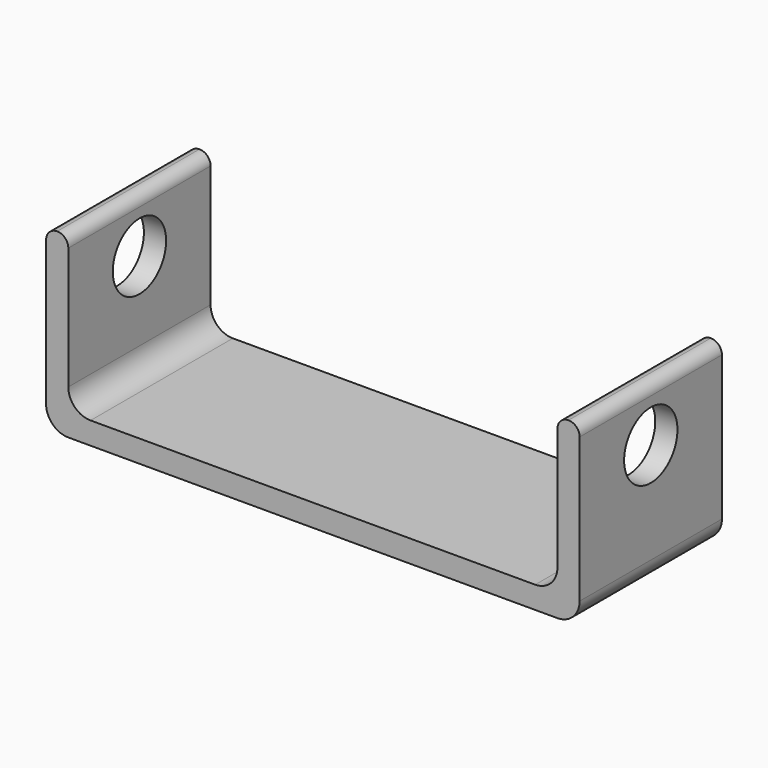
from build123d import *

# Parameters (mm, degrees)
F1_DEPTH = 25.4
F2_R     = 6.35
F3_R     = 3.17499
F4_R     = 9.525
F5_DEPTH = 152.401


# Not quite as in the source:
# - a fillet or chamfer is up to 0.001 mm smaller than in the source, because OpenCascade refuses the exact size


with BuildPart() as f1:
    # F0 (on Front) → F1 (new body, symmetric)
    with BuildSketch(Plane.XZ):
        Polygon((-76.2, 0), (0, 0), (76.2, 0), (76.2, 50.8), (69.85, 50.8), (69.85, 6.35), (0, 6.35), (-69.85, 6.35), (-69.85, 50.8), (-76.2, 50.8), align=None)
    extrude(amount=F1_DEPTH, both=True)

    # F2
    f2_edges = [f1.edges().sort_by_distance(p)[0] for p in [
        (-69.85, 0, 6.35),
        (69.85, 0, 6.35),
        (76.2, 0, 0),
        (-76.2, 0, 0),
    ]]
    fillet(f2_edges, radius=F2_R)

    # F3 (radius 3.175 in the source; OpenCascade refuses exactly that, so slightly less here)
    f3_edges = [f1.edges().sort_by_distance(p)[0] for p in [
        (-69.85, 0, 50.8),
        (-76.2, 0, 50.8),
        (69.85, 0, 50.8),
        (76.2, 0, 50.8),
    ]]
    fillet(f3_edges, radius=F3_R)

    # F4 (on face) → F5 (cut, through all)
    with BuildSketch(Plane(origin=(-76.2, 0, 0), x_dir=(0, -1, 0), z_dir=(-1, 0, 0))):
        with Locations((0, 35.2541096509)):
            Circle(F4_R)
    extrude(amount=-F5_DEPTH, mode=Mode.SUBTRACT)


solid = f1.part
